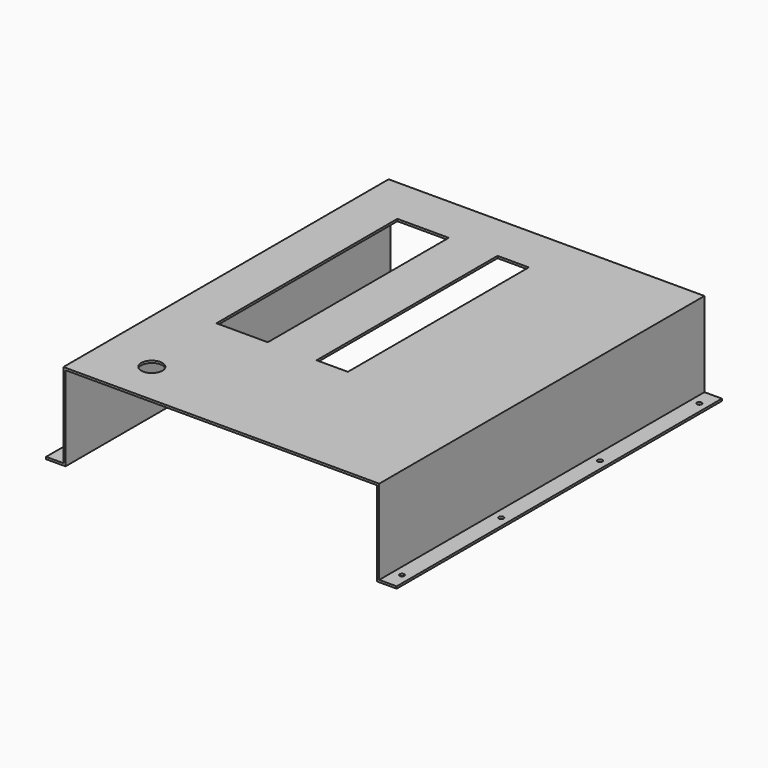
from build123d import *

# Parameters (mm, degrees)
F1_DEPTH = 609.092
F3_W     = 76.98
F3_H     = 338.836
F3_W_2   = 46.863
F4_DEPTH = 25.4
F6_R     = 15.875
F7_DEPTH = 25.4
F8_D     = 7.14375


# Not quite as in the source:
# - a length typed as a fraction of an inch, garbled in the dataset ("3 / 203.2 mm" for 3/8 in), is restored


with BuildPart() as f1:
    # F0 (on Front) → F1 (new body)
    with BuildSketch(Plane.XZ):
        Polygon((0, -3.175), (0, 0), (-26.162, 0), (-26.162, 126.873), (-499.364, 126.873), (-499.364, 0), (-525.272, 0), (-525.272, -3.175), (-496.189, -3.175), (-496.189, 123.698), (-29.337, 123.698), (-29.337, -3.175), align=None)
    extrude(amount=F1_DEPTH)

    # F3 (on face) → F4 (cut)
    with BuildSketch(Plane.XY.offset(126.873)):
        with Locations((-390.262, -241.3)):
            Rectangle(F3_W, F3_H)
        with Locations((-255.262, -241.3)):
            Rectangle(F3_W_2, F3_H)
    extrude(amount=-F4_DEPTH, mode=Mode.SUBTRACT)

    # F6 (on face) → F7 (cut)
    with BuildSketch(Plane.XY.offset(126.873)):
        with Locations((-418.846, -544.068)):
            Circle(F6_R)
    extrude(amount=-F7_DEPTH, mode=Mode.SUBTRACT)

    # F8 (through all)
    with Locations(Plane.XY):
        with Locations((-512.318, -25.908), (-512.318, -212.09), (-512.318, -397.002), (-512.318, -582.93), (-12.954, -582.93), (-12.954, -397.002), (-12.954, -212.09), (-12.954, -25.908)):
            Hole(F8_D / 2)


solid = f1.part
